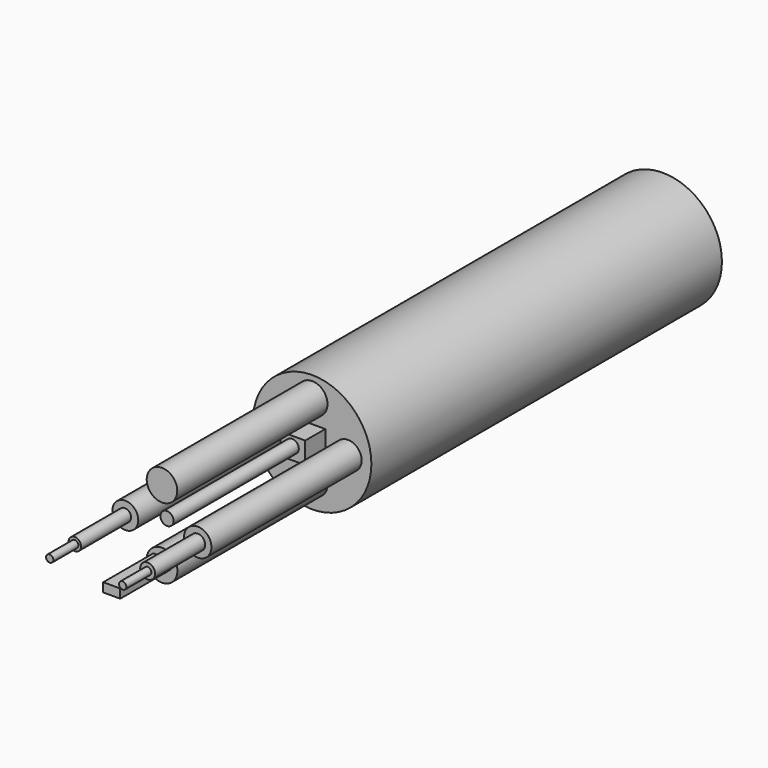
from build123d import *

# Parameters (mm, degrees)
F0_R      = 24.0021072249
F1_DEPTH  = 177.8
F2_R      = 5.2565656239
F2_R_2    = 5.5580260463
F3_DEPTH  = 76.2
F4_R      = 2.5394375709
F4_R_2    = 3.0260152953
F5_DEPTH  = 25.4
F6_R      = 1.4824915772
F6_R_2    = 1.4854629447
F7_DEPTH  = 12.7
F8_W      = 9.9838948809
F8_H      = 8.7704055477
F9_DEPTH  = 10.16
F10_R     = 2.6763905771
F11_DEPTH = 63.5
F12_R     = 6.2569040354
F13_DEPTH = 76.2
F14_W     = 6.9022711832
F14_H     = 3.66242975
F15_DEPTH = 25.4
F16_R     = 6.2007059651
F17_DEPTH = 76.2


# Not quite as in the source:
# - a length typed as a fraction of an inch, garbled in the dataset ("3 / 203.2 mm" for 3/8 in), is restored


with BuildPart() as f1:
    # F0 (on Front) → F1 (new body)
    with BuildSketch(Plane.XZ):
        Circle(F0_R)
    extrude(amount=F1_DEPTH)

    # F2 (on face) → F3 (join)
    with BuildSketch(Plane.XZ.offset(177.8)):
        with Locations((-14.8806795478, 0)):
            Circle(F2_R)
        with Locations((14.4999595359, 0)):
            Circle(F2_R_2)
    extrude(amount=F3_DEPTH)

    # F4 (on face) → F5 (join)
    with BuildSketch(Plane.XZ.offset(254)):
        with Locations((-15.0723066181, 0)):
            Circle(F4_R)
        with Locations((14.4999595359, 0)):
            Circle(F4_R_2)
    extrude(amount=F5_DEPTH)

    # F6 (on face) → F7 (join)
    with BuildSketch(Plane.XZ.offset(279.4)):
        with Locations((-15.0723066181, 0)):
            Circle(F6_R)
        with Locations((14.5250931382, 0)):
            Circle(F6_R_2)
    extrude(amount=F7_DEPTH)

    # F8 (on face) → F9 (join)
    with BuildSketch(Plane.XZ.offset(177.8)):
        with Locations((0.2944918815, 2.0464671543)):
            Rectangle(F8_W, F8_H)
    extrude(amount=F9_DEPTH)

    # F10 (on face) → F11 (join)
    with BuildSketch(Plane.XZ.offset(187.96)):
        with Locations((0, 2.6763908099)):
            Circle(F10_R)
    extrude(amount=F11_DEPTH)

    # F12 (on face) → F13 (join)
    with BuildSketch(Plane.XZ.offset(177.8)):
        with Locations((0, -12.9593666643)):
            Circle(F12_R)
    extrude(amount=F13_DEPTH)

    # F14 (on face) → F15 (join)
    with BuildSketch(Plane.XZ.offset(254)):
        with Locations((-0.0704309205, -11.6916019469)):
            Rectangle(F14_W, F14_H)
    extrude(amount=F15_DEPTH)

    # F16 (on face) → F17 (join)
    with BuildSketch(Plane.XZ.offset(177.8)):
        with Locations((0, 15.626385808)):
            Circle(F16_R)
    extrude(amount=F17_DEPTH)


solid = f1.part
